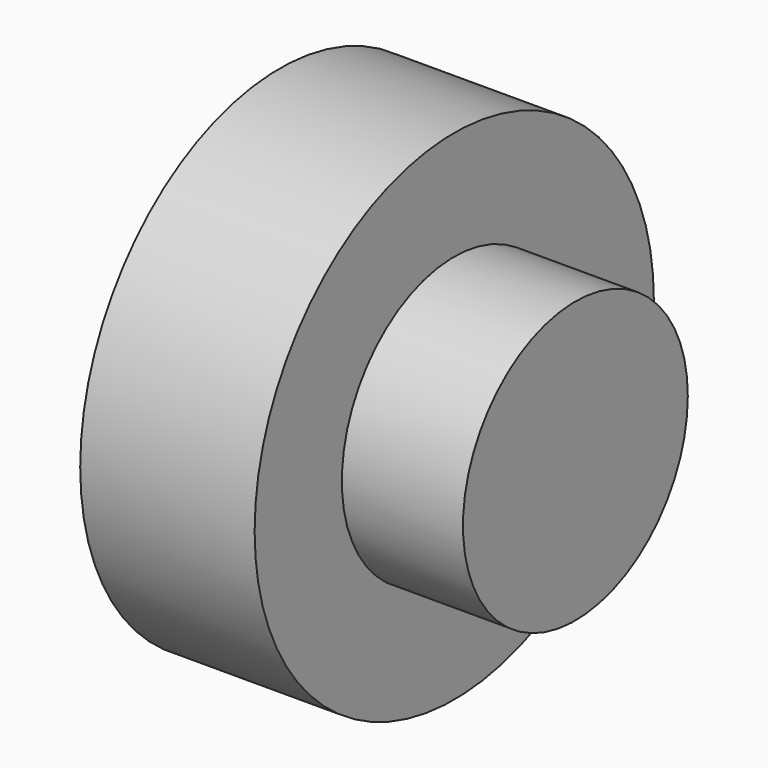
from build123d import *

# Parameters (mm, degrees)
F0_R     = 103
F1_DEPTH = 36
F2_R     = 58
F3_DEPTH = 50
F4_R     = 58
F5_DEPTH = 15
F6_R     = 9.5
F7_DEPTH = 45
F8_W     = 6
F8_H     = 4
F9_DEPTH = 35
F10_R    = 2.9999


# Not quite as in the source:
# - a fillet or chamfer is up to 0.001 mm smaller than in the source, because OpenCascade refuses the exact size


with BuildPart() as f1:
    # F0 (on Right) → F1 (new body, symmetric)
    with BuildSketch(Plane.YZ):
        Circle(F0_R)
    extrude(amount=F1_DEPTH, both=True)

    # F2 (on face) → F3 (join)
    with BuildSketch(Plane.YZ.offset(36)):
        Circle(F2_R)
    extrude(amount=F3_DEPTH)

    # F4 (on face) → F5 (join)
    with BuildSketch(Plane(origin=(-36, 0, 0), x_dir=(0, -1, 0), z_dir=(-1, 0, 0))):
        Circle(F4_R)
    extrude(amount=F5_DEPTH)

    # F6 (on face) → F7 (join)
    with BuildSketch(Plane(origin=(-51, 0, 0), x_dir=(0, -1, 0), z_dir=(-1, 0, 0))):
        Circle(F6_R)
    extrude(amount=F7_DEPTH)

    # F8 (on face) → F9 (cut)
    with BuildSketch(Plane(origin=(-96, 0, 0), x_dir=(0, -1, 0), z_dir=(-1, 0, 0))):
        with Locations((0, 9.5)):
            Rectangle(F8_W, F8_H)
    extrude(amount=-F9_DEPTH, mode=Mode.SUBTRACT)

    # F10 (radius 3 in the source; OpenCascade refuses exactly that, so slightly less here)
    f10_edges = [f1.edges().sort_by_distance(p)[0] for p in [
        (-61, 3, 8.256939),
        (-61, -3, 8.256939),
    ]]
    fillet(f10_edges, radius=F10_R)


solid = f1.part
